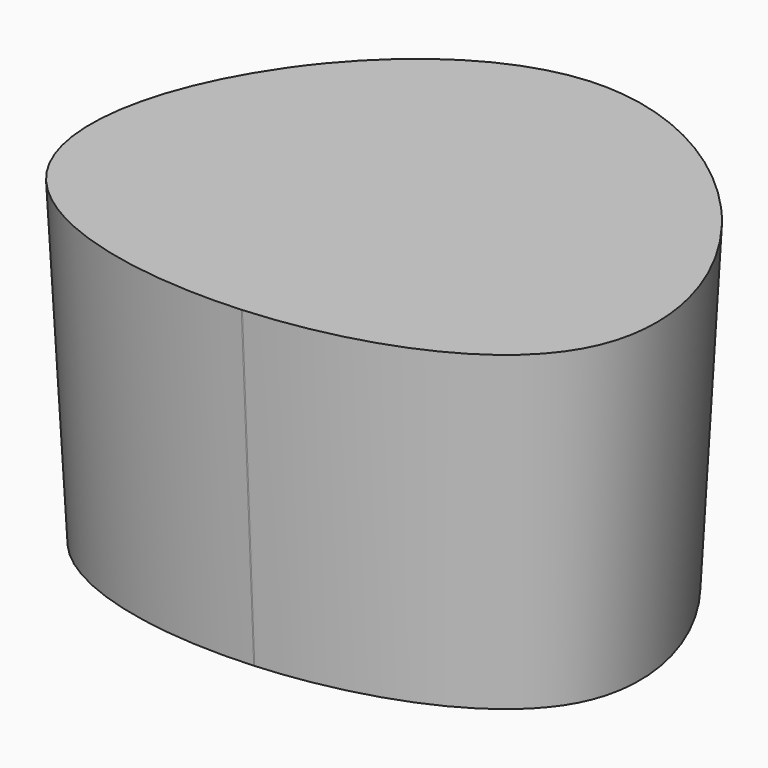
from build123d import *

# Parameters (mm, degrees)
F1_DEPTH = 50
F1_TAPER = -3


# Not quite as in the source:
# - the program builds the solid bodies; features that only make, move or delete a surface that nothing else refers to are left out


with BuildPart() as f1:
    # F0 (on Top) → F1 (new body)
    with BuildSketch(Plane.XY):
        with BuildLine():
            add(Edge.make_bspline(
                [(0, 29.4209048152), (24.3763025366, 30.9887818451), (79.4951551623, -38.8729245738), (-70.587758018, -48.7950519549), (-24.4365075818, 27.8491554135), (0, 29.4209048152)],
                knots=[0, 0, 0, 0, 0.3248021011, 0.6743956966, 1, 1, 1, 1], degree=3))
        make_face()
    extrude(amount=F1_DEPTH, taper=F1_TAPER)


solid = f1.part
